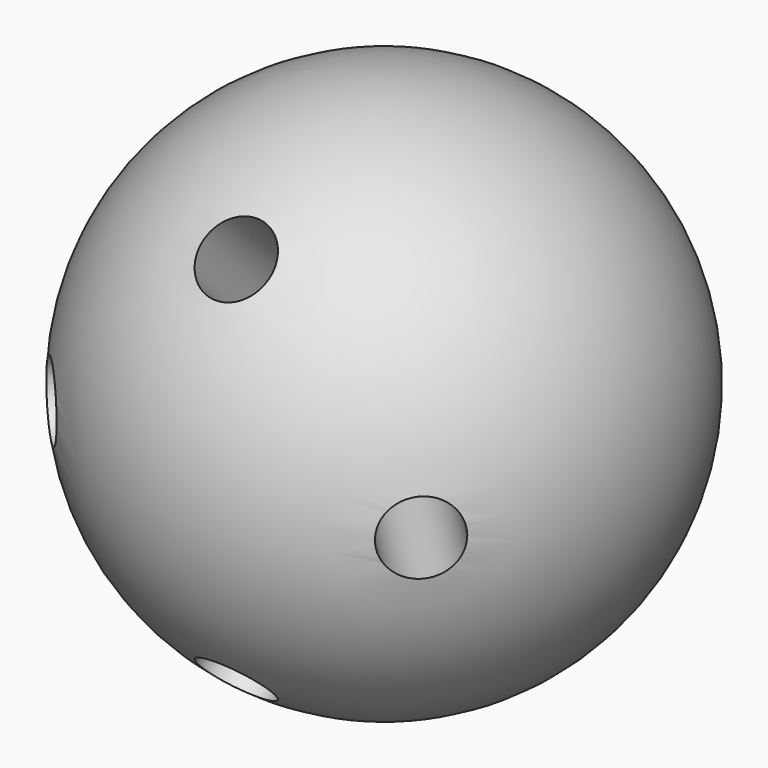
from build123d import *

# Parameters (mm, degrees)
F5_R            = 2.75
F6_DEPTH        = 11
F6_COPIES_COUNT = 4


# Not quite as in the source:
# - a pattern or mirror of a feature is missing from the dataset's text; its kind, count and spacing are read off the source's solid


with BuildPart() as f2:
    # F1 (on Front) → F2 (revolve)
    with BuildSketch(Plane.XZ):
        with BuildLine():
            ThreePointArc((0, 20), (-20, 0), (0, -20))
            Line((0, -20), (0, 20))
        make_face()
    revolve(axis=Axis((0, 0, 0), (0, 0, -1)))

    # F5 (on line) → F6 (cut)
    with BuildSketch(Plane(origin=(14.1421356237, -14.1421356237, 0), x_dir=(0.7071067812, 0.7071067812, 0), z_dir=(0.7071067812, -0.7071067812, 0))):
        Circle(F5_R)
    f6 = extrude(amount=-F6_DEPTH, mode=Mode.SUBTRACT)

    # F6_copies: F6 ×4 about axis
    f6_copies_axis = Axis((0, 0, 0), (0, 1, 0))
    for i in range(1, F6_COPIES_COUNT):
        add(f6.rotate(f6_copies_axis, i * 360 / F6_COPIES_COUNT), mode=Mode.SUBTRACT)


solid = f2.part
